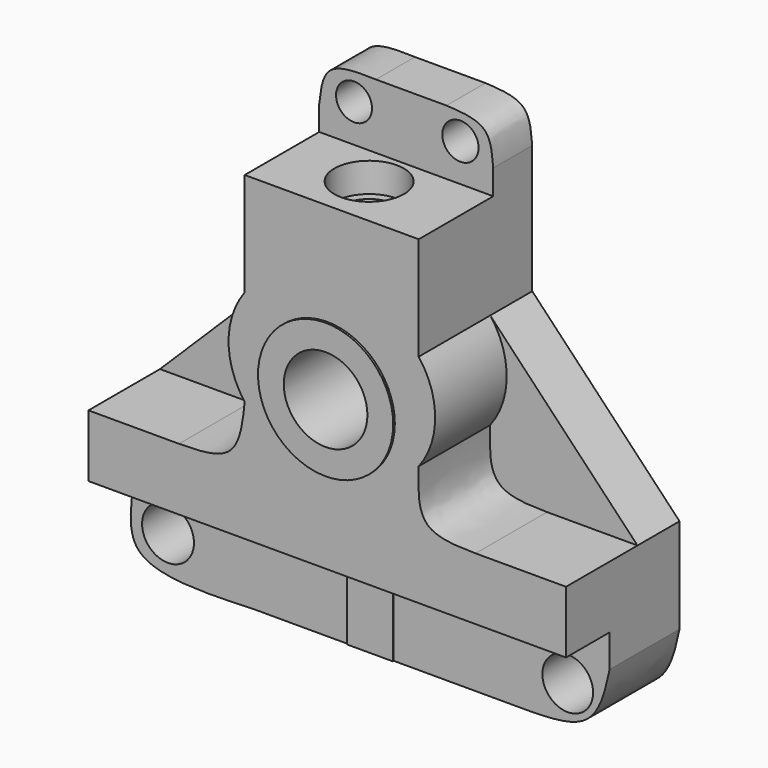
from build123d import *

# Parameters (mm, degrees)
F1_DEPTH  = 31.52012
F0_R      = 3.9989944529
F0_R_2    = 4.0304935081
F2_DEPTH  = 10.8295
F3_DEPTH  = 11.66704
F0_R_3    = 9.2896599899
F4_DEPTH  = 31.97776
F6_R      = 7.7262681343
F6_R_2    = 5.87306791
F7_DEPTH  = 7.37838
F9_DEPTH  = 23.31858
F0_R_4    = 5.7595758306
F0_R_5    = 5.6310949549
F10_DEPTH = 19.41152
F0_W      = 10.16
F0_H      = 21.1746012493
F11_DEPTH = 19.65592


# Not quite as in the source:
# - a feature names something its author has since deleted; it is built from what else it names
# - the program builds the solid bodies; features that only make, move or delete a surface that nothing else refers to are left out


with BuildPart() as f1:
    # F0 (on Front) → F1 (new body)
    with BuildSketch(Plane.XZ):
        with BuildLine():
            Line((-32.945703147, 0), (-53.0377118984, 0))
            Line((-53.0377118984, 0), (-53.0377118984, -13.8332377828))
            Line((-53.0377118984, -13.8332377828), (-5.08, -13.8332377828))
            Line((-5.08, -13.8332377828), (5.08, -13.8332377828))
            Line((5.08, -13.8332377828), (53.0377118984, -13.8332377828))
            Line((53.0377118984, -13.8332377828), (53.0377118984, 0))
            Line((53.0377118984, 0), (32.945703147, 0))
            add(Edge.make_bspline(
                [(32.945703147, 0), (28.5647447129, 0.0625927983), (19.8735598839, 0.1867678132), (20.1720018391, 8.6992646442), (20.3200084018, 12.9208741543)],
                knots=[0, 0, 0, 0, 0.5040691828, 1, 1, 1, 1], degree=3))
            ThreePointArc((20.3200084018, 12.9208741543), (23.9781287511, 23.6330514006), (20.3200084018, 34.345228647))
            Line((20.3200084018, 34.345228647), (20.3200084018, 57.3156722881))
            Line((20.3200084018, 57.3156722881), (-18.3321793468, 57.3156722881))
            Line((-18.3321793468, 57.3156722881), (-18.3321793468, 34.345228647))
            ThreePointArc((-18.3321793468, 34.345228647), (-21.9102829622, 23.6330514006), (-18.3321793468, 12.9208741543))
            add(Edge.make_bspline(
                [(-32.945703147, 0), (-28.5122837396, 0.0592468916), (-19.728591274, 0.176629532), (-18.7947032642, 8.6996856696), (-18.3321793468, 12.9208741543)],
                knots=[0, 0, 0, 0, 0.5047329952, 1, 1, 1, 1], degree=3))
        make_face()
        with BuildLine():
            ThreePointArc((6.2648822412, 33.191720318), (12.6390408842, 27.6514544893), (15.0142637131, 19.5469643528))
            ThreePointArc((15.0142637131, 19.5469643528), (-7.6843579979, 6.6481753784), (-7.1484956716, 32.75026411))
            ThreePointArc((-7.1484956716, 32.75026411), (-0.4938765731, 34.5531031225), (6.2648822412, 33.191720318))
        make_face(mode=Mode.SUBTRACT)
    extrude(amount=F1_DEPTH)

    # F0 (on Front) → F2 (join)
    with BuildSketch(Plane.XZ):
        with BuildLine():
            Line((-18.3321793468, 62.8374100943), (-18.3321793468, 57.3156722881))
            Line((-18.3321793468, 57.3156722881), (20.3200084018, 57.3156722881))
            Line((20.3200084018, 57.3156722881), (20.3200084018, 62.8374100943))
            add(Edge.make_bspline(
                [(20.3200084018, 62.8374100943), (20.1052749574, 65.5197235908), (19.6543576651, 71.15229537), (13.2786405866, 71.4934853371), (9.9391337225, 71.6721956254)],
                knots=[0, 0, 0, 0, 0.4762147029, 1, 1, 1, 1], degree=3))
            Line((9.9391337225, 71.6721956254), (-5.7426103852, 71.6721956254))
            add(Edge.make_bspline(
                [(-18.3321793468, 62.8374100943), (-18.0134703448, 65.7269619482), (-17.326155356, 71.9584530192), (-9.7862501304, 71.772123737), (-5.7426103852, 71.6721956254)],
                knots=[0, 0, 0, 0, 0.4637015156, 1, 1, 1, 1], degree=3))
        make_face()
        with Locations((-10.6017430574, 65.7269619482)):
            Circle(F0_R, mode=Mode.SUBTRACT)
        with Locations((13.0313078181, 65.7087189627)):
            Circle(F0_R_2, mode=Mode.SUBTRACT)
    extrude(amount=F2_DEPTH)

    # F0 (on Front) → F3 (join)
    with BuildSketch(Plane.XZ):
        with BuildLine():
            Line((-18.3321793468, 34.345228647), (-53.0377118984, 0))
            Line((-53.0377118984, 0), (-32.945703147, 0))
            add(Edge.make_bspline(
                [(-32.945703147, 0), (-28.5122837396, 0.0592468916), (-19.728591274, 0.176629532), (-18.7947032642, 8.6996856696), (-18.3321793468, 12.9208741543)],
                knots=[0, 0, 0, 0, 0.5047329952, 1, 1, 1, 1], degree=3))
            ThreePointArc((-18.3321793468, 12.9208741543), (-21.9102829622, 23.6330514006), (-18.3321793468, 34.345228647))
        make_face()
        with BuildLine():
            Line((53.0377118984, 0), (20.3200084018, 34.345228647))
            ThreePointArc((20.3200084018, 34.345228647), (23.9781287511, 23.6330514006), (20.3200084018, 12.9208741543))
            add(Edge.make_bspline(
                [(32.945703147, 0), (28.5647447129, 0.0625927983), (19.8735598839, 0.1867678132), (20.1720018391, 8.6992646442), (20.3200084018, 12.9208741543)],
                knots=[0, 0, 0, 0, 0.5040691828, 1, 1, 1, 1], degree=3))
            Line((32.945703147, 0), (53.0377118984, 0))
        make_face()
    extrude(amount=F3_DEPTH)

    # F0 (on Front) → F4 (join)
    with BuildSketch(Plane.XZ):
        with BuildLine():
            ThreePointArc((-7.1484956716, 32.75026411), (-7.6843579979, 6.6481753784), (15.0142637131, 19.5469643528))
            ThreePointArc((15.0142637131, 19.5469643528), (12.6390408842, 27.6514544893), (6.2648822412, 33.191720318))
            ThreePointArc((6.2648822412, 33.191720318), (-0.4938765731, 34.5531031225), (-7.1484956716, 32.75026411))
        make_face()
        with Locations((0, 19.5469643528)):
            Circle(F0_R_3, mode=Mode.SUBTRACT)
    extrude(amount=F4_DEPTH)

    # F6 (on offset) → F7 (cut)
    with BuildSketch(Plane.XY.offset(50.8)):
        with Locations((0, -19.8897793889)):
            Circle(F6_R)
        with Locations((0, -19.8897793889)):
            Circle(F6_R_2, mode=Mode.SUBTRACT)
    extrude(amount=F7_DEPTH, mode=Mode.SUBTRACT)

    # F9 (cut): a face of the model
    f9_faces = [f1.faces().sort_by_distance(p)[0] for p in [
        (0, -19.8897793889, 57.3156722881),
    ]]
    extrude(f9_faces, amount=-F9_DEPTH, mode=Mode.SUBTRACT)

    # F0 (on Front) → F10 (join)
    with BuildSketch(Plane.XZ):
        with BuildLine():
            Line((-5.08, -13.8332377828), (-53.0377118984, -13.8332377828))
            Line((-53.0377118984, -13.8332377828), (-53.0377118984, -21.0930503504))
            add(Edge.make_bspline(
                [(-53.0377118984, -21.0930503504), (-53.4005944702, -25.2780429079), (-54.7251608325, -36.2581171884), (-35.7792689312, -35.346119388), (-25.8417483085, -35.0078390322)],
                knots=[0, 0, 0, 0, 0.3981682681, 1, 1, 1, 1], degree=3))
            Line((-25.8417483085, -35.0078390322), (-5.08, -35.0078390322))
            Line((-5.08, -35.0078390322), (-5.08, -13.8332377828))
        make_face()
        with Locations((-45.0574053683, -26.3939229293)):
            Circle(F0_R_4, mode=Mode.SUBTRACT)
        with BuildLine():
            Line((53.0377118984, -13.8332377828), (5.08, -13.8332377828))
            Line((5.08, -13.8332377828), (5.08, -35.0078390322))
            Line((5.08, -35.0078390322), (35.7808830812, -35.0078390322))
            add(Edge.make_bspline(
                [(53.0377118984, -21.0930503504), (52.1158724207, -25.6188280404), (49.8115979989, -34.1905224475), (41.3452471932, -34.893061815), (35.7808830812, -35.0078390322)],
                knots=[0, 0, 0, 0, 0.4907243677, 1, 1, 1, 1], degree=3))
            Line((53.0377118984, -21.0930503504), (53.0377118984, -13.8332377828))
        make_face()
        with Locations((43.7321887989, -26.8356617858)):
            Circle(F0_R_5, mode=Mode.SUBTRACT)
    extrude(amount=F10_DEPTH)

    # F0 (on Front) → F11 (join)
    with BuildSketch(Plane.XZ):
        with Locations((0, -24.4205384075)):
            Rectangle(F0_W, F0_H)
    extrude(amount=F11_DEPTH)


solid = f1.part
